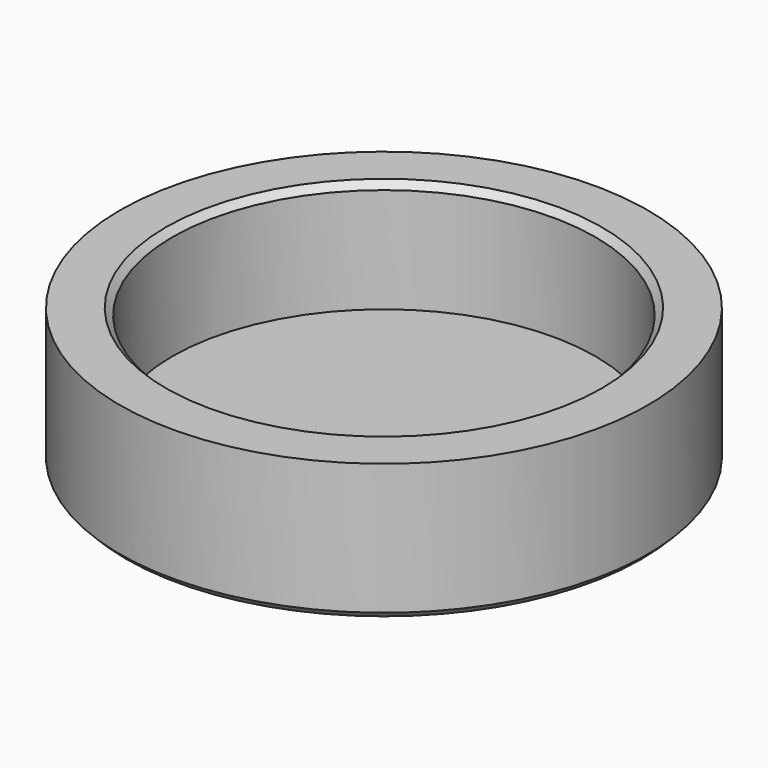
from build123d import *

# Parameters (mm, degrees)
F2_SIZE      = 0.2
F3_TEXT_SIZE = 14.8779192297
F4_DEPTH     = 0.2


# Not quite as in the source:
# - Text() gives the source's letters only with a copy of the font that has no kerning and outlines rounded to 1/6400 em; it was checked with that copy


with BuildPart() as f1:
    # F0 (on Front) → F1 (revolve)
    with BuildSketch(Plane.XZ):
        Polygon((0, -0.8), (0, 0), (-6.45, 0), (-6.45, 3.4), (-8.05, 3.4), (-8.05, -0.8), align=None)
    revolve(axis=Axis((0, 0, -0.4), (0, 0, 1)))

    # F2
    f2_edges = [f1.edges().sort_by_distance(p)[0] for p in [
        (8.05, 0, -0.8),
        (6.45, 0, 3.4),
    ]]
    chamfer(f2_edges, length=F2_SIZE)

    # F3 (on face) → F4 (cut)
    with BuildSketch(Plane(origin=(0, 0, -0.8), x_dir=(1, 0, 0), z_dir=(0, 0, -1))):
        with Locations((-5.3932457208, -5.3560509227)):
            Text('R', F3_TEXT_SIZE, font='Open Sans', font_style=FontStyle.BOLD, text_align=(TextAlign.LEFT, TextAlign.BOTTOM))
    extrude(amount=-F4_DEPTH, mode=Mode.SUBTRACT)


solid = f1.part
